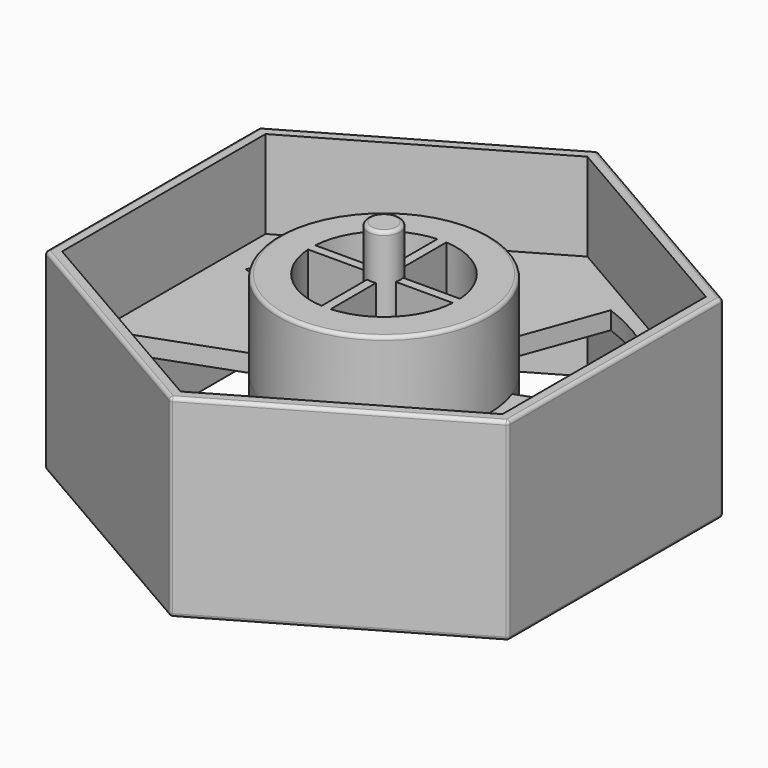
from build123d import *
from build123d import SkipClean  # not in build123d's __all__

# Parameters (mm, degrees)
F1_DEPTH      = 27.5
F2_R          = 15
F3_DEPTH      = 12.5
F4_R          = 15
F5_DEPTH      = 12.5
F7_DEPTH      = 27.501
F8_R          = 2.29
F9_DEPTH      = 6.25
F9_DEPTH_BACK = 34
F10_R         = 0.5
F12_DEPTH     = 21.251


with BuildPart() as f1:
    # F0 (on Top) → F1 (new body)
    with BuildSketch(Plane.XY):
        Polygon((32.9089653438, 19), (0, 38), (-32.9089653438, 19), (-32.9089653438, -19), (0, -38), (32.9089653438, -19), align=None)
    extrude(amount=F1_DEPTH)

    # F2 (on face) → F3 (cut)
    with BuildSketch(Plane.XY.offset(27.5)):
        Polygon((0, -36.1293851278), (31.2889653438, -18.0646925639), (31.2889653438, 18.0646925639), (0, 36.1293851278), (-31.2889653438, 18.0646925639), (-31.2889653438, -18.0646925639), align=None)
        Circle(F2_R, mode=Mode.SUBTRACT)
    extrude(amount=-F3_DEPTH, mode=Mode.SUBTRACT)

    # F4 (on face) → F5 (cut)
    with BuildSketch(Plane(origin=(0, 0, 0), x_dir=(1, 0, 0), z_dir=(0, 0, -1))):
        Polygon((0, -36.1293851278), (31.2889653438, -18.0646925639), (31.2889653438, 18.0646925639), (0, 36.1293851278), (-31.2889653438, 18.0646925639), (-31.2889653438, -18.0646925639), align=None)
        Circle(F4_R, mode=Mode.SUBTRACT)
    extrude(amount=-F5_DEPTH, mode=Mode.SUBTRACT)

    # F6 (on face) → F7 (cut, through all)
    with BuildSketch(Plane(origin=(0, 0, 0), x_dir=(1, 0, 0), z_dir=(0, 0, -1))):
        with BuildLine():
            Line((0.64, 0.64), (10.2800972758, 0.64))
            ThreePointArc((10.2800972758, 0.64), (7.2831998462, 7.2831998462), (0.64, 10.2800972758))
            Line((0.64, 10.2800972758), (0.64, 0.64))
        make_face()
        with BuildLine():
            Line((0.64, -0.64), (0.64, -10.2800972758))
            ThreePointArc((0.64, -10.2800972758), (7.2831998462, -7.2831998462), (10.2800972758, -0.64))
            Line((10.2800972758, -0.64), (0.64, -0.64))
        make_face()
        with BuildLine():
            ThreePointArc((-10.2800972758, -0.64), (-7.2831998462, -7.2831998462), (-0.64, -10.2800972758))
            Line((-0.64, -10.2800972758), (-0.64, -0.64))
            Line((-0.64, -0.64), (-10.2800972758, -0.64))
        make_face()
        with BuildLine():
            ThreePointArc((-0.64, 10.2800972758), (-7.2831998462, 7.2831998462), (-10.2800972758, 0.64))
            Line((-10.2800972758, 0.64), (-0.64, 0.64))
            Line((-0.64, 0.64), (-0.64, 10.2800972758))
        make_face()
    extrude(amount=-F7_DEPTH, mode=Mode.SUBTRACT)

    # F8 (on face) → F9 (join, two sides)
    with BuildSketch(Plane(origin=(0, 0, 0), x_dir=(1, 0, 0), z_dir=(0, 0, -1))) as f9_sk:
        Circle(F8_R)
    extrude(amount=F9_DEPTH)
    extrude(f9_sk.sketch, amount=-F9_DEPTH_BACK)

    # F10
    f10_edges = [f1.edges().sort_by_distance(p)[0] for p in [
        (-15, 0, 0),
        (-15, 0, 27.5),
        (-2.29, 0, -6.25),
        (-2.29, 0, 34),
        (-32.908965, 19, 13.75),
        (-32.908965, -19, 13.75),
        (-32.908965, 0, 0),
        (-32.908965, 0, 27.5),
        (0, 38, 13.75),
        (-16.454483, 28.5, 0),
        (-16.454483, 28.5, 27.5),
        (32.908965, 19, 13.75),
        (16.454483, 28.5, 0),
        (16.454483, 28.5, 27.5),
        (32.908965, -19, 13.75),
        (32.908965, 0, 0),
        (32.908965, 0, 27.5),
        (0, -38, 13.75),
        (16.454483, -28.5, 0),
        (16.454483, -28.5, 27.5),
        (-16.454483, -28.5, 0),
        (-16.454483, -28.5, 27.5),
    ]]
    fillet(f10_edges, radius=F10_R)

    # F11 (on face) → F12 (cut, through all)
    with BuildSketch(Plane.XY.offset(15)):
        with BuildLine():
            Line((-14.0953893118, -5.1303021499), (-27.6843442082, -10.076277247))
            ThreePointArc((-27.6843442082, -10.076277247), (-20.83211796, -20.83211796), (-10.076277247, -27.6843442082))
            Line((-10.076277247, -27.6843442082), (-5.1303021499, -14.0953893118))
            ThreePointArc((-5.1303021499, -14.0953893118), (-10.6066017178, -10.6066017178), (-14.0953893118, -5.1303021499))
        make_face()
        with BuildLine():
            Line((-27.6843442082, 10.076277247), (-14.0953893118, 5.1303021499))
            ThreePointArc((-14.0953893118, 5.1303021499), (-10.6066017178, 10.6066017178), (-5.1303021499, 14.0953893118))
            Line((-5.1303021499, 14.0953893118), (-10.076277247, 27.6843442082))
            ThreePointArc((-10.076277247, 27.6843442082), (-20.83211796, 20.83211796), (-27.6843442082, 10.076277247))
        make_face()
        with BuildLine():
            Line((10.076277247, 27.6843442082), (5.1303021499, 14.0953893118))
            ThreePointArc((5.1303021499, 14.0953893118), (10.6066017178, 10.6066017178), (14.0953893118, 5.1303021499))
            Line((14.0953893118, 5.1303021499), (27.6843442082, 10.076277247))
            ThreePointArc((27.6843442082, 10.076277247), (20.83211796, 20.83211796), (10.076277247, 27.6843442082))
        make_face()
        with BuildLine():
            ThreePointArc((14.0953893118, -5.1303021499), (10.6066017178, -10.6066017178), (5.1303021499, -14.0953893118))
            Line((5.1303021499, -14.0953893118), (10.076277247, -27.6843442082))
            ThreePointArc((10.076277247, -27.6843442082), (20.83211796, -20.83211796), (27.6843442082, -10.076277247))
            Line((27.6843442082, -10.076277247), (14.0953893118, -5.1303021499))
        make_face()
    with SkipClean():  # cleaning this boolean's faces spoils the solid; the shape is the same uncleaned
        extrude(amount=-F12_DEPTH, mode=Mode.SUBTRACT)


solid = f1.part
